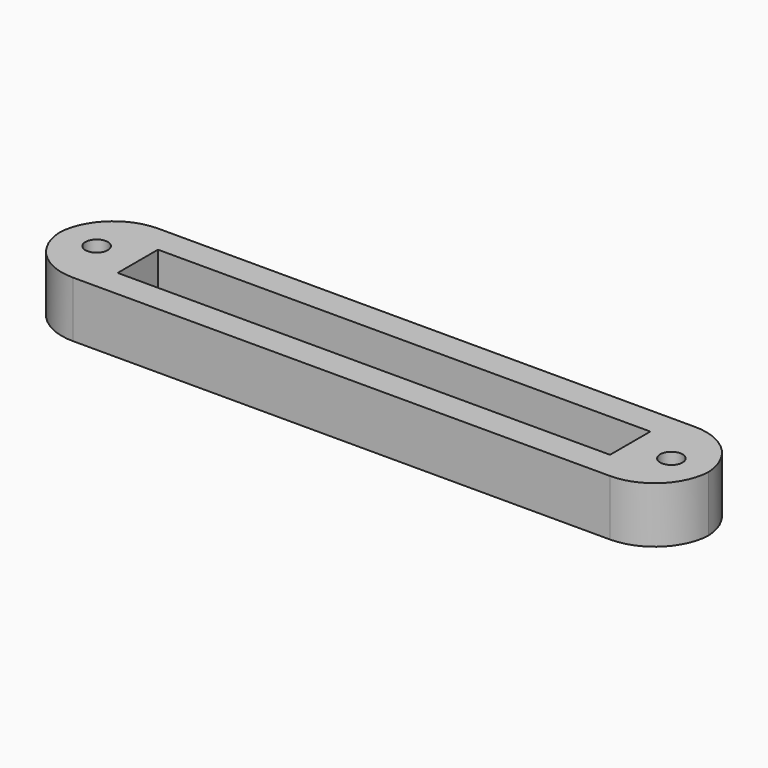
from build123d import *

# Parameters (mm, degrees)
F0_W        = 58
F0_H        = 9.5
F0_R        = 1
F0_W_2      = 44
F0_H_2      = 4.5
F1_DEPTH    = 5
F2_T1_DEPTH = 30


# Not quite as in the source:
# - a fillet or chamfer that OpenCascade refuses, or shapes differently, is made with other operations: its cross-section is extruded or revolved along the edge and cut away or added


with BuildPart() as f1:
    # F0 (on Top) → F1 (new body)
    with BuildSketch(Plane.XY):
        Rectangle(F0_W, F0_H)
        with Locations((-25.6825946271, 0)):
            Circle(F0_R, mode=Mode.SUBTRACT)
        Rectangle(F0_W_2, F0_H_2, mode=Mode.SUBTRACT)
        with Locations((25.6825946271, 0)):
            Circle(F0_R, mode=Mode.SUBTRACT)
    extrude(amount=F1_DEPTH)

    # F2: fillet of radius 5 on 4 edges, made by hand

    # F2_s2 → F2_t1 (cut)
    with BuildSketch(Plane.XY.offset(-12.5)):
        with BuildLine():
            ThreePointArc((24, -4.75), (27.5355339059, -3.2855339059), (29, 0.25))
            Line((29, 0.25), (29, -4.75))
            Line((29, -4.75), (24, -4.75))
        make_face()
        with BuildLine():
            ThreePointArc((29, -0.25), (27.5355339059, 3.2855339059), (24, 4.75))
            Line((24, 4.75), (29, 4.75))
            Line((29, 4.75), (29, -0.25))
        make_face()
        with BuildLine():
            ThreePointArc((-24, 4.75), (-27.5355339059, 3.2855339059), (-29, -0.25))
            Line((-29, -0.25), (-29, 4.75))
            Line((-29, 4.75), (-24, 4.75))
        make_face()
        with BuildLine():
            ThreePointArc((-24, -4.75), (-27.5355339059, -3.2855339059), (-29, 0.25))
            Line((-29, 0.25), (-29, -4.75))
            Line((-29, -4.75), (-24, -4.75))
        make_face()
    extrude(amount=F2_T1_DEPTH, mode=Mode.SUBTRACT)


solid = f1.part
